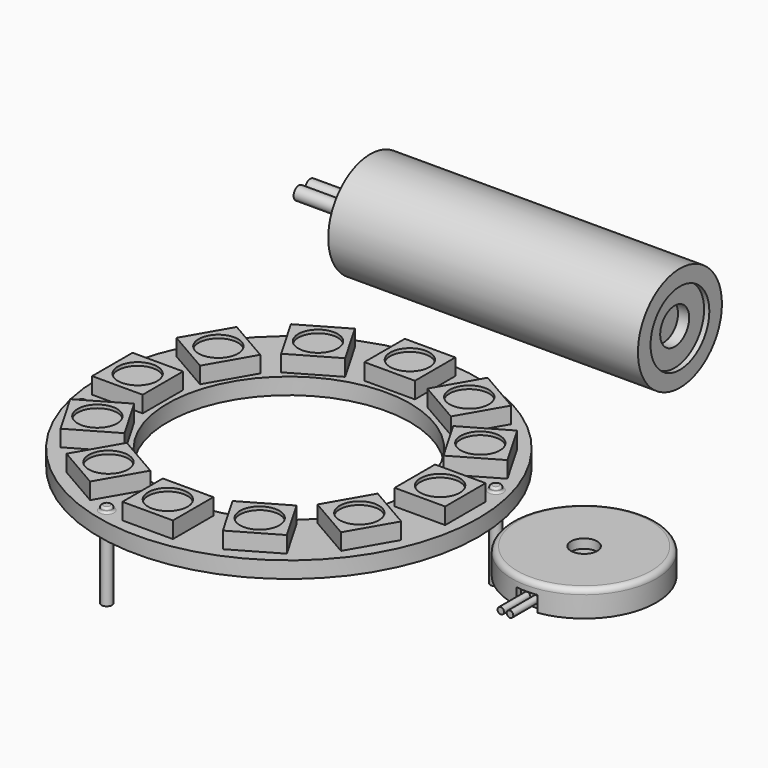
from build123d import *

# Parameters (mm, degrees)
F0_R          = 18.3515
F0_R_2        = 0.508
F0_R_3        = 11.7348
F1_DEPTH      = 1.5875
F2_W          = 4.8895
F2_H          = 4.8895
F2_R          = 1.905
F3_DEPTH      = 1.5875
F4_DEPTH      = 1.27
F5_DEPTH      = 6.35
F5_DEPTH_BACK = 2.032
F6_R          = 0.2032
F7_R          = 6.985
F8_DEPTH      = 2.54
F9_R          = 0.508
F10_R         = 1.27
F11_DEPTH     = 0.889
F13_START     = 6.35
F12_W         = 2.032
F12_H         = 1.524
F13_DEPTH     = 1.27
F14_R         = 0.3175
F15_DEPTH     = 3.175
F16_R         = 5.08
F17_DEPTH     = 14.986
F18_R         = 1.7526
F19_DEPTH     = 1.5875
F18_R_2       = 3.556
F20_DEPTH     = 0.508
F21_R         = 0.635
F22_DEPTH     = 6.35


with BuildPart() as f1:
    # F0 (on Top) → F1 (new body)
    with BuildSketch(Plane.XY):
        Circle(F0_R)
        with Locations((-4.4210175189, -16.4994620018)):
            Circle(F0_R_2, mode=Mode.SUBTRACT)
        with Locations((-16.4994620018, -4.4210175189)):
            Circle(F0_R_2, mode=Mode.SUBTRACT)
        Circle(F0_R_3, mode=Mode.SUBTRACT)
        with Locations((16.4994620018, 4.4210175189)):
            Circle(F0_R_2, mode=Mode.SUBTRACT)
        with Locations((4.4210175189, 16.4994620018)):
            Circle(F0_R_2, mode=Mode.SUBTRACT)
    extrude(amount=F1_DEPTH)

    # F2 (on face) → F3 (join)
    with BuildSketch(Plane.XY.offset(1.5875)):
        with Locations((0, 14.63675)):
            Rectangle(F2_W, F2_H)
        with Locations((0, 14.63675)):
            Circle(F2_R, mode=Mode.SUBTRACT)
        Polygon((-6.4235343941, 16.0153879347), (-10.6579656059, 13.5706379347), (-8.2132156059, 9.3362067229), (-3.9787843941, 11.7809567229), align=None)
        with Locations((-7.318375, 12.6757973288)):
            Circle(F2_R, mode=Mode.SUBTRACT)
        Polygon((-13.5706379347, 10.6579656059), (-16.0153879347, 6.4235343941), (-11.7809567229, 3.9787843941), (-9.3362067229, 8.2132156059), align=None)
        with Locations((-12.6757973288, 7.318375)):
            Circle(F2_R, mode=Mode.SUBTRACT)
        with Locations((-14.63675, 0)):
            Rectangle(F2_W, F2_H)
        with Locations((-14.63675, 0)):
            Circle(F2_R, mode=Mode.SUBTRACT)
        Polygon((-16.0153879347, -6.4235343941), (-13.5706379347, -10.6579656059), (-9.3362067229, -8.2132156059), (-11.7809567229, -3.9787843941), align=None)
        with Locations((-12.6757973288, -7.318375)):
            Circle(F2_R, mode=Mode.SUBTRACT)
        Polygon((-10.6579656059, -13.5706379347), (-6.4235343941, -16.0153879347), (-3.9787843941, -11.7809567229), (-8.2132156059, -9.3362067229), align=None)
        with Locations((-7.318375, -12.6757973288)):
            Circle(F2_R, mode=Mode.SUBTRACT)
        with Locations((0, -14.63675)):
            Rectangle(F2_W, F2_H)
        with Locations((0, -14.63675)):
            Circle(F2_R, mode=Mode.SUBTRACT)
        Polygon((6.4235343941, -16.0153879347), (10.6579656059, -13.5706379347), (8.2132156059, -9.3362067229), (3.9787843941, -11.7809567229), align=None)
        with Locations((7.318375, -12.6757973288)):
            Circle(F2_R, mode=Mode.SUBTRACT)
        Polygon((13.5706379347, -10.6579656059), (16.0153879347, -6.4235343941), (11.7809567229, -3.9787843941), (9.3362067229, -8.2132156059), align=None)
        with Locations((12.6757973288, -7.318375)):
            Circle(F2_R, mode=Mode.SUBTRACT)
        with Locations((14.63675, 0)):
            Rectangle(F2_W, F2_H)
        with Locations((14.63675, 0)):
            Circle(F2_R, mode=Mode.SUBTRACT)
        Polygon((16.0153879347, 6.4235343941), (13.5706379347, 10.6579656059), (9.3362067229, 8.2132156059), (11.7809567229, 3.9787843941), align=None)
        with Locations((12.6757973288, 7.318375)):
            Circle(F2_R, mode=Mode.SUBTRACT)
        Polygon((10.6579656059, 13.5706379347), (6.4235343941, 16.0153879347), (3.9787843941, 11.7809567229), (8.2132156059, 9.3362067229), align=None)
        with Locations((7.318375, 12.6757973288)):
            Circle(F2_R, mode=Mode.SUBTRACT)
    extrude(amount=F3_DEPTH)

    # F4 (add): faces of the model
    f4_faces = [f1.faces().sort_by_distance(p)[0] for p in [
        (0, 14.63675, 1.5875),
        (7.318375, 12.6757973288, 1.5875),
        (12.6757973288, 7.318375, 1.5875),
        (14.63675, 0, 1.5875),
        (12.6757973288, -7.318375, 1.5875),
        (7.318375, -12.6757973288, 1.5875),
        (0, -14.63675, 1.5875),
        (-7.318375, -12.6757973288, 1.5875),
        (-12.6757973288, -7.318375, 1.5875),
        (-14.63675, 0, 1.5875),
        (-12.6757973288, 7.318375, 1.5875),
        (-7.318375, 12.6757973288, 1.5875),
    ]]
    extrude(f4_faces, amount=F4_DEPTH)

    # F0 (on Top) → F5 (join, two sides)
    with BuildSketch(Plane.XY) as f5_sk:
        with Locations((-4.4210175189, -16.4994620018)):
            Circle(F0_R_2)
        with Locations((-16.4994620018, -4.4210175189)):
            Circle(F0_R_2)
        with Locations((16.4994620018, 4.4210175189)):
            Circle(F0_R_2)
    extrude(amount=-F5_DEPTH)
    extrude(f5_sk.sketch, amount=F5_DEPTH_BACK)

    # F6
    f6_edges = [f1.edges().sort_by_distance(p)[0] for p in [
        (15.991462, 4.421018, 1.5875),
        (15.991462, 4.421018, 2.032),
        (-17.007462, -4.421018, 2.032),
        (-4.929018, -16.499462, 2.032),
        (-17.007462, -4.421018, 1.5875),
        (-4.929018, -16.499462, 1.5875),
    ]]
    fillet(f6_edges, radius=F6_R)


with BuildPart() as f8:
    # F7 (on Top) → F8 (new body)
    with BuildSketch(Plane.XY):
        with Locations((28.575, 0)):
            Circle(F7_R)
    extrude(amount=F8_DEPTH)

    # F9
    f9_edges = [f8.edges().sort_by_distance(p)[0] for p in [
        (21.59, 0, 2.54),
    ]]
    fillet(f9_edges, radius=F9_R)

    # F10 (on face) → F11 (cut)
    with BuildSketch(Plane.XY.offset(2.54)):
        with Locations((28.575, 0)):
            Circle(F10_R)
    extrude(amount=-F11_DEPTH, mode=Mode.SUBTRACT)

    # F12 (on Front) → F13 (cut)
    with BuildSketch(Plane.XZ.offset(F13_START)):
        with Locations((28.575, 0.762)):
            Rectangle(F12_W, F12_H)
    extrude(amount=F13_DEPTH, mode=Mode.SUBTRACT)

    # F14 (on face) → F15 (join)
    with BuildSketch(Plane.XZ.offset(6.35)):
        with Locations((28.1305, 0.762)):
            Circle(F14_R)
        with Locations((29.0195, 0.762)):
            Circle(F14_R)
    extrude(amount=F15_DEPTH)


with BuildPart() as f17:
    # F16 (on Right) → F17 (new body, symmetric)
    with BuildSketch(Plane.YZ):
        with Locations((28.575, 5.08)):
            Circle(F16_R)
    extrude(amount=F17_DEPTH, both=True)

    # F18 (on face) → F19 (cut)
    with BuildSketch(Plane.YZ.offset(14.986)):
        with Locations((28.575, 5.08)):
            Circle(F18_R)
    extrude(amount=-F19_DEPTH, mode=Mode.SUBTRACT)

    # F18 (on face) → F20 (cut)
    with BuildSketch(Plane.YZ.offset(14.986)):
        with Locations((28.575, 5.08)):
            Circle(F18_R_2)
        with Locations((28.575, 5.08)):
            Circle(F18_R, mode=Mode.SUBTRACT)
    extrude(amount=-F20_DEPTH, mode=Mode.SUBTRACT)

    # F21 (on face) → F22 (join)
    with BuildSketch(Plane(origin=(-14.986, 0, 0), x_dir=(0, -1, 0), z_dir=(-1, 0, 0))):
        with Locations((-29.2735, 5.08)):
            Circle(F21_R)
        with Locations((-27.8765, 5.08)):
            Circle(F21_R)
    extrude(amount=F22_DEPTH)

    # F24 (on offset) → F25 (revolve)
    with BuildSketch(Plane.XY.offset(5.08)):
        Polygon((-16.5735, 29.9085), (-16.5735, 28.575), (-14.986, 28.575), (-14.986, 31.877), align=None)
    revolve(axis=Axis((-15.77975, 28.575, 5.08), (1, 0, 0)))


solid = Compound([f1.part, f8.part, f17.part])
